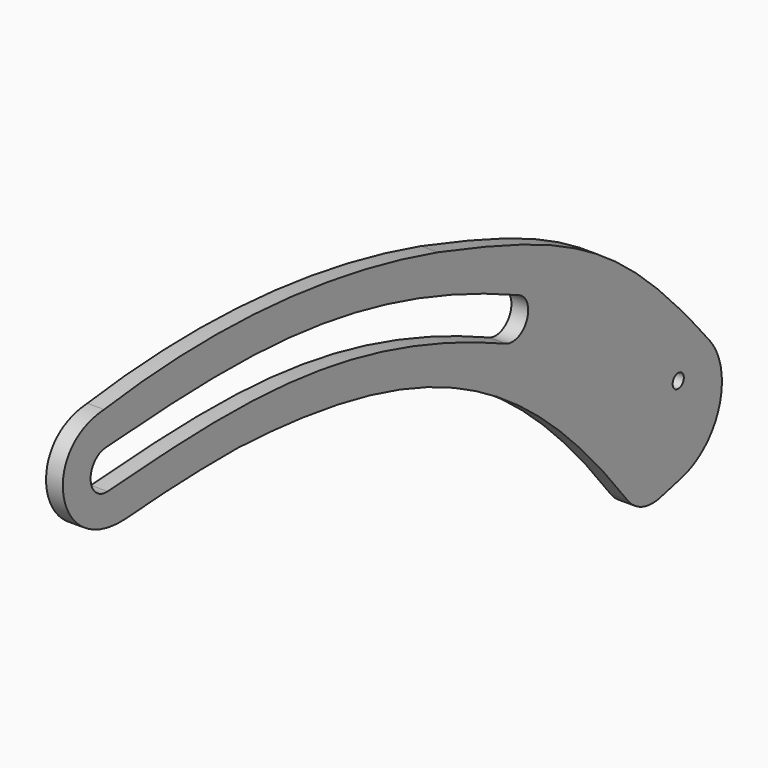
from build123d import *

# Parameters (mm, degrees)
F0_R     = 2.65
F1_DEPTH = 6.35


# Not quite as in the source:
# - the dataset's text gives a spline's control points without its knots; the knots are read off the source's solid


with BuildPart() as f1:
    # F0 (on Right) → F1 (new body)
    with BuildSketch(Plane.YZ):
        with BuildLine():
            Line((261.9483946854, -115.7954504994), (272.1252628725, -113.2826431827))
            ThreePointArc((272.1252628725, -113.2826431827), (289.8889070688, -96.7979835608), (285.3293778213, -72.9966863058))
            add(Edge.make_bspline(
                [(156.7577297495, 8.6854864661), (221.6098067843, -11.5913002759), (243.8542047817, -23.2805241602), (285.3293778213, -72.9966863058)],
                knots=[0, 0, 0, 0, 161.109408384, 161.109408384, 161.109408384, 161.109408384], degree=3))
            ThreePointArc((156.7577297495, 8.6854864661), (78.4544562182, 22.8327000089), (-1.0815155301, 20.4714514424))
            add(Edge.make_bspline(
                [(9.3677433569, -20.0565137491), (-24.1417251725, -22.0444979462), (-32.3005802929, 18.4173323214), (-1.0815155301, 20.4714514424)],
                knots=[0, 0, 0, 0, 41.8533508079, 41.8533508079, 41.8533508079, 41.8533508079], degree=3))
            ThreePointArc((9.3677433569, -20.0565137491), (35.7155181109, -18.446549817), (62.1091524383, -18.0302742562))
            add(Edge.make_bspline(
                [(246.4764264248, -110.3954762242), (199.3983001687, -49.3749203985), (153.2148223134, -21.8351859288), (62.1091524383, -18.0302742562)],
                knots=[8.5665161252, 8.5665161252, 8.5665161252, 8.5665161252, 214.9819028362, 214.9819028362, 214.9819028362, 214.9819028362], degree=3))
            ThreePointArc((246.4764264248, -110.3954762242), (253.4098300896, -115.3950112589), (261.9483946854, -115.7954504994))
        make_face()
        with Locations((270.459651947, -80.3557708859)):
            Circle(F0_R, mode=Mode.SUBTRACT)
        with BuildLine():
            add(Edge.make_bspline(
                [(0.5223238355, -7.4817897465), (16.1473752008, -6.3909629477), (38.554977526, -4.9102528421), (67.8852104449, -4.9151730534), (90.0179145686, -6.311914144), (112.710472254, -9.5107891223), (136.3998847667, -14.9334158805), (161.5182791316, -23.0182515025), (179.4931658657, -30.4824293605), (188.8537865884, -34.8081819283)],
                knots=[0, 0, 0, 0, 0.25, 0.375, 0.5, 0.625, 0.75, 0.875, 1, 1, 1, 1], degree=3))
            ThreePointArc((0.5223238355, -7.4817897465), (-7.4817897465, -0.5223238355), (-0.5223238355, 7.4817897465))
            add(Edge.make_bspline(
                [(-0.5223238355, 7.4817897465), (15.1365957215, 8.5749809747), (37.8985666734, 10.087587055), (68.3190062607, 10.0887299467), (91.5209291721, 8.6278442992), (115.443956431, 5.2569378265), (140.4104220259, -0.4597325437), (166.7475341855, -8.9410706921), (185.448960915, -16.7105004187), (195.1462134116, -21.1918180717)],
                knots=[0, 0, 0, 0, 0.25, 0.375, 0.5, 0.625, 0.75, 0.875, 1, 1, 1, 1], degree=3))
            ThreePointArc((195.1462134116, -21.1918180717), (198.8081819283, -31.1462134116), (188.8537865884, -34.8081819283))
        make_face(mode=Mode.SUBTRACT)
    extrude(amount=F1_DEPTH)


solid = f1.part
